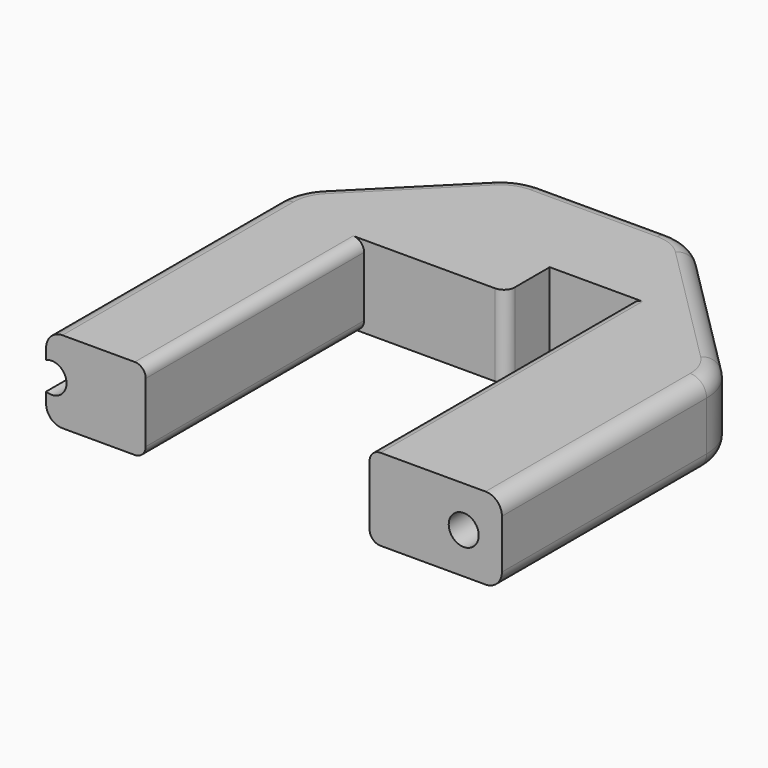
from build123d import *

# Parameters (mm, degrees)
F1_DEPTH    = 80
F0_W        = 20.5
F0_H        = 15
F0_W_2      = 5.5
F2_DEPTH    = 30
F0_W_3      = 15
F3_DEPTH    = 20
F4_T1_DEPTH = 123.2356797549
F4_T3_DEPTH = 123.2356797549
F5_T1_DEPTH = 164.157613302
F6_R        = 10
F7_R        = 2
F8_R        = 3


# Not quite as in the source:
# - a fillet or chamfer that OpenCascade refuses, or shapes differently, is made with other operations: its cross-section is extruded or revolved along the edge and cut away or added


with BuildPart() as f1:
    # F0 (on Front) → F1 (new body)
    with BuildSketch(Plane.XZ):
        with BuildLine():
            Line((-20.5, 15), (-38.75, 15))
            Line((-38.75, 15), (-38.75, 10.0617376915))
            ThreePointArc((-38.75, 10.0617376915), (-36.1987907943, 9.7707377656), (-35, 7.5))
            ThreePointArc((-35, 7.5), (-36.1987907943, 5.2292622344), (-38.75, 4.9382623085))
            Line((-38.75, 4.9382623085), (-38.75, 0))
            Line((-38.75, 0), (-20.5, 0))
            Line((-20.5, 0), (-20.5, 15))
        make_face()
    extrude(amount=F1_DEPTH)

    # F0 (on Front) → F2 (join)
    with BuildSketch(Plane.XZ):
        with Locations((-10.25, 7.5)):
            Rectangle(F0_W, F0_H)
        with Locations((2.75, 7.5)):
            Rectangle(F0_W_2, F0_H)
    extrude(amount=F2_DEPTH)



with BuildPart() as f1b:
    # F0 (on Front) → F1, piece 2 (new body)
    with BuildSketch(Plane.XZ):
        with BuildLine():
            Line((38.75, 15), (20.5, 15))
            Line((20.5, 15), (20.5, 0))
            Line((20.5, 0), (38.75, 0))
            Line((38.75, 0), (38.75, 4.9382623085))
            ThreePointArc((38.75, 4.9382623085), (35, 7.5), (38.75, 10.0617376915))
            Line((38.75, 10.0617376915), (38.75, 15))
        make_face()
        with BuildLine():
            Line((44.75, 15), (38.75, 15))
            Line((38.75, 15), (38.75, 10.0617376915))
            ThreePointArc((38.75, 10.0617376915), (40.0207377656, 9.0512092057), (40.5, 7.5))
            ThreePointArc((40.5, 7.5), (40.0207377656, 5.9487907943), (38.75, 4.9382623085))
            Line((38.75, 4.9382623085), (38.75, 0))
            Line((38.75, 0), (44.75, 0))
            Line((44.75, 0), (44.75, 15))
        make_face()
    extrude(amount=F1_DEPTH)


with BuildPart() as f1_1:
    add(f1.part)

    add(f1b.part)  # F3 merges F1b
    # F0 (on Front) → F3 (join)
    with BuildSketch(Plane.XZ):
        with Locations((13, 7.5)):
            Rectangle(F0_W_3, F0_H)
    extrude(amount=F3_DEPTH)

    # F4: chamfer of 23 on 2 edges, made by hand

    # F4_s2 → F4_t1 (cut)
    with BuildSketch(Plane.XY.offset(-59.1487087232)):
        Polygon((-15.75, 0), (-38.75, -23), (-38.75, 0), align=None)
    extrude(amount=F4_T1_DEPTH, mode=Mode.SUBTRACT)

    # F4_s4 → F4_t3 (cut)
    with BuildSketch(Plane.XY.offset(-49.0869710317)):
        Polygon((-15.75, 0), (-38.75, -23), (-38.75, 0), align=None)
    extrude(amount=F4_T3_DEPTH, mode=Mode.SUBTRACT)

    # F5: chamfer of 29 on 1 edges, made by hand

    # F5_s2 → F5_t1 (cut)
    with BuildSketch(Plane.XY.offset(-74.578806651)):
        Polygon((15.75, 0), (44.75, -29), (44.75, 0), align=None)
    extrude(amount=F5_T1_DEPTH, mode=Mode.SUBTRACT)

    # F6
    f6_edges = [f1_1.edges().sort_by_distance(p)[0] for p in [
        (15.75, 0, 7.5),
        (-15.75, 0, 7.5),
        (44.75, -29, 7.5),
        (-38.75, -23, 2.469131),
        (-38.75, -23, 12.530869),
    ]]
    fillet(f6_edges, radius=F6_R)

    # F7
    f7_edges = [f1_1.edges().sort_by_distance(p)[0] for p in [
        (20.5, -50, 15),
        (20.5, -50, 0),
        (-20.5, -55, 15),
        (-20.5, -55, 0),
        (5.5, -30, 7.5),
    ]]
    fillet(f7_edges, radius=F7_R)

    # F8
    f8_edges = [f1_1.edges().sort_by_distance(p)[0] for p in [
        (-38.75, -53.571068, 15),
        (-37.988795, -23.315301, 15),
        (-27.25, -11.5, 15),
        (-15.434699, -0.761205, 15),
        (0, 0, 15),
        (15.434699, -0.761205, 15),
        (30.25, -14.5, 15),
        (43.988795, -29.315301, 15),
        (44.75, -56.571068, 15),
        (44.75, -56.571068, 0),
        (43.988795, -29.315301, 0),
        (-38.75, -53.571068, 0),
        (-37.988795, -23.315301, 0),
        (-27.25, -11.5, 0),
        (-15.434699, -0.761205, 0),
        (0, 0, 0),
        (15.434699, -0.761205, 0),
        (30.25, -14.5, 0),
    ]]
    fillet(f8_edges, radius=F8_R)


solid = f1_1.part
